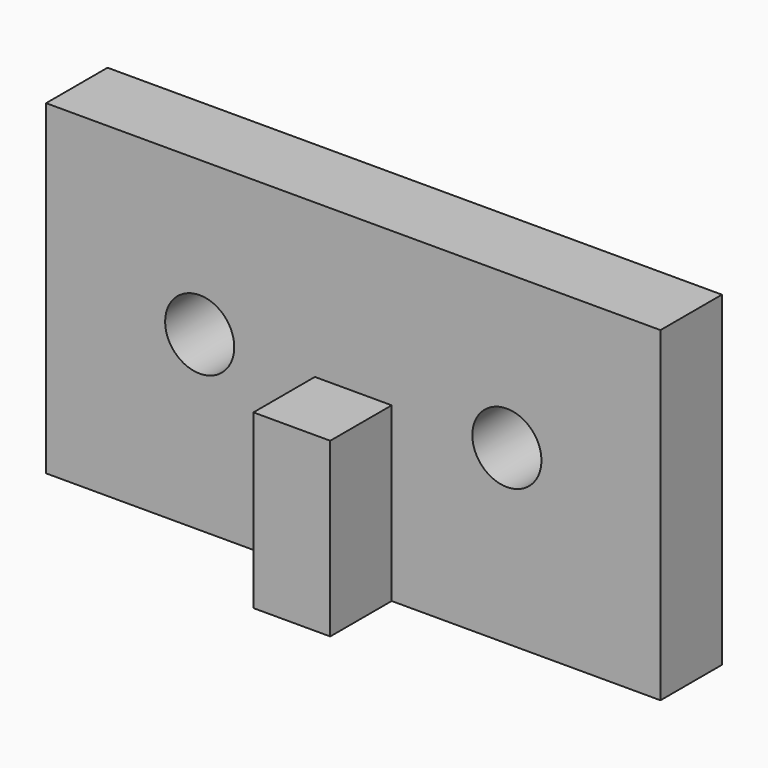
from build123d import *

# Parameters (mm, degrees)
F0_W     = 17.5
F0_H     = 21.2181335688
F0_W_2   = 5
F1_DEPTH = 5
F2_W     = 5
F2_H     = 11.2181335688
F3_DEPTH = 5
F4_D     = 4.5
F4_DEPTH = 17
F4_TIP   = 1.3519363928


with BuildPart() as f1:
    # F0 (on Front) → F1 (new body)
    with BuildSketch(Plane.XZ):
        with Locations((-11.25, 49.3909332156)):
            Rectangle(F0_W, F0_H)
        with Locations((0, 49.3909332156)):
            Rectangle(F0_W_2, F0_H)
        with Locations((11.25, 49.3909332156)):
            Rectangle(F0_W, F0_H)
    extrude(amount=F1_DEPTH)

    # F2 (on face) → F3 (join)
    with BuildSketch(Plane.XZ.offset(5)):
        with Locations((0, 44.3909332156)):
            Rectangle(F2_W, F2_H)
    extrude(amount=F3_DEPTH)

    # F4
    with Locations(Plane(origin=(0, 0, 0), x_dir=(1, 0, 0), z_dir=(0, 1, 0))):
        with Locations((10, -50), (-10, -50)):
            Hole(F4_D / 2, depth=F4_DEPTH)
            with Locations((0, 0, -(F4_DEPTH + F4_TIP / 2))):  # 118° drill point
                Cone(0, F4_D / 2, F4_TIP, mode=Mode.SUBTRACT)


solid = f1.part
